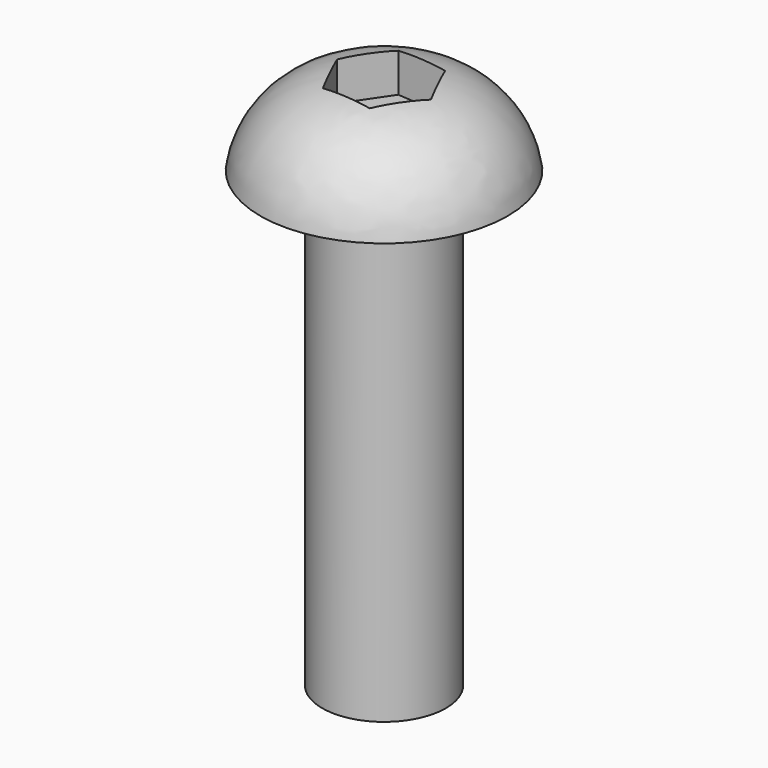
from build123d import *

# Parameters (mm, degrees)
F0_R     = 3
F0_R_2   = 1.5
F1_DEPTH = 2
F2_DEPTH = 11
F6_DEPTH = 1.5


# Not quite as in the source:
# - a fillet or chamfer that OpenCascade refuses, or shapes differently, is made with other operations: its cross-section is extruded or revolved along the edge and cut away or added


with BuildPart() as f1:
    # F0 (on Top) → F1 (new body)
    with BuildSketch(Plane.XY):
        Circle(F0_R)
        Circle(F0_R_2, mode=Mode.SUBTRACT)
        Circle(F0_R_2)
    extrude(amount=F1_DEPTH)

    # F0 (on Top) → F2 (join)
    with BuildSketch(Plane.XY):
        Circle(F0_R_2)
    extrude(amount=-F2_DEPTH)

    # F3: fillet of radius 2.3417871555 on 1 edges, made by hand

    # F3_s1 → F3_t2 (revolve, cut)
    with BuildSketch(Plane.XZ):
        with BuildLine():
            ThreePointArc((3, 0), (2.2135791593, 1.4308323542), (0.6832892667, 2))
            Line((0.6832892667, 2), (3, 2))
            Line((3, 2), (3, 0))
        make_face()
    revolve(axis=Axis((0, 0, 2), (0, 0, 1)), mode=Mode.SUBTRACT)

    # F5 (on offset) → F6 (cut)
    with BuildSketch(Plane.XY.offset(2.5)):
        Polygon((0.5268892093, -1.0919650915), (1.209114114, -0.0896831055), (0.6822249046, 1.002281986), (-0.5268892093, 1.0919650915), (-1.209114114, 0.0896831055), (-0.6822249046, -1.002281986), align=None)
    extrude(amount=-F6_DEPTH, mode=Mode.SUBTRACT)


solid = f1.part
